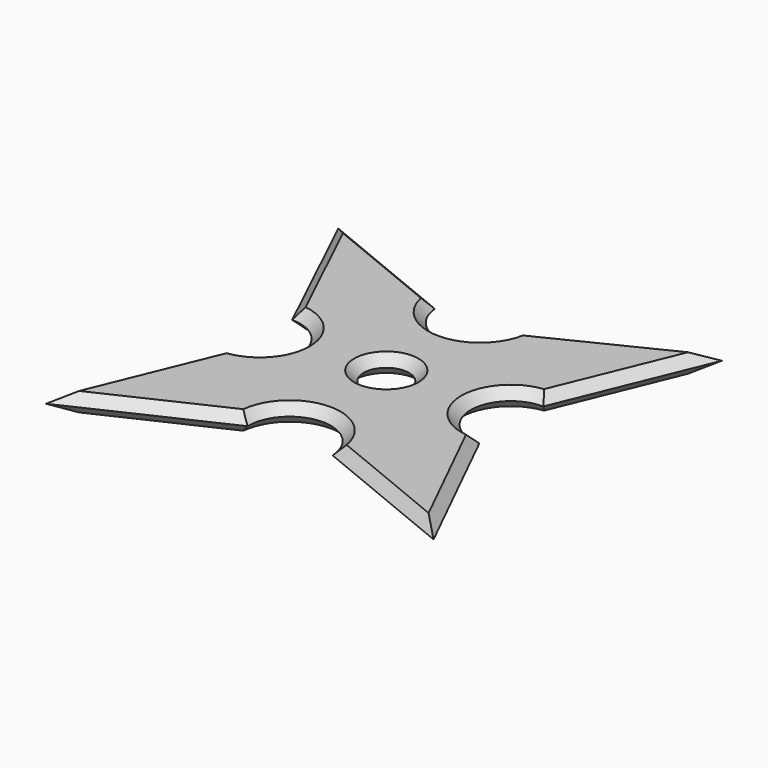
from build123d import *

# Parameters (mm, degrees)
F0_R     = 5.9800521353
F1_DEPTH = 5
F2_SIZE  = 2.49999


# Not quite as in the source:
# - a fillet or chamfer is up to 0.001 mm smaller than in the source, because OpenCascade refuses the exact size


with BuildPart() as f1:
    # F0 (on Top) → F1 (new body)
    with BuildSketch(Plane.XY):
        with BuildLine():
            Line((27.7623478323, 49.0298643708), (11.5457307547, 9.5314830542))
            Line((11.5457307547, 9.5314830542), (50.2365343273, 27.6623163372))
            ThreePointArc((50.2365343273, 27.6623163372), (60.7722385086, 38.8133091708), (72.0498927169, 28.4132986261))
            Line((72.0498927169, 28.4132986261), (111.7447488987, 12.1160160238))
            Line((111.7447488987, 12.1160160238), (92.3213660153, 51.5245050192))
            ThreePointArc((92.3213660153, 51.5245050192), (81.6154488918, 62.0616839697), (92.3213660153, 72.5988629201))
            Line((92.3213660153, 72.5988629201), (108.314871788, 111.5538179874))
            Line((108.314871788, 111.5538179874), (69.9733346701, 92.6563069494))
            ThreePointArc((69.9733346701, 92.6563069494), (58.8159662766, 82.4438797358), (47.6585978831, 92.6563069494))
            Line((47.6585978831, 92.6563069494), (9.7151305526, 108.2345321774))
            Line((9.7151305526, 108.2345321774), (27.7623478323, 70.4347789288))
            ThreePointArc((27.7623478323, 70.4347789288), (38.47065847, 59.7323216498), (27.7623478323, 49.0298643708))
        make_face()
        with Locations((60, 61.2126085907)):
            Circle(F0_R, mode=Mode.SUBTRACT)
    extrude(amount=F1_DEPTH)

    # F2 (size 2.5 in the source; OpenCascade refuses exactly that, so slightly less here)
    f2_edges = [f1.edges().sort_by_distance(p)[0] for p in [
        (28.686864, 100.44542, 5),
        (18.738739, 89.334656, 5),
        (38.470658, 59.732322, 5),
        (19.654039, 29.280674, 5),
        (30.891133, 18.5969, 5),
        (60.772239, 38.813309, 5),
        (91.897321, 20.264657, 5),
        (102.033057, 31.820261, 5),
        (81.615449, 62.061684, 5),
        (100.318119, 92.07634, 5),
        (89.144103, 102.105062, 5),
        (58.815966, 82.44388, 5),
        (54.019948, 61.212609, 5),
        (28.686864, 100.44542, 0),
        (18.738739, 89.334656, 0),
        (38.470658, 59.732322, 0),
        (19.654039, 29.280674, 0),
        (30.891133, 18.5969, 0),
        (60.772239, 38.813309, 0),
        (91.897321, 20.264657, 0),
        (102.033057, 31.820261, 0),
        (81.615449, 62.061684, 0),
        (100.318119, 92.07634, 0),
        (89.144103, 102.105062, 0),
        (58.815966, 82.44388, 0),
        (54.019948, 61.212609, 0),
    ]]
    chamfer(f2_edges, length=F2_SIZE)


solid = f1.part
